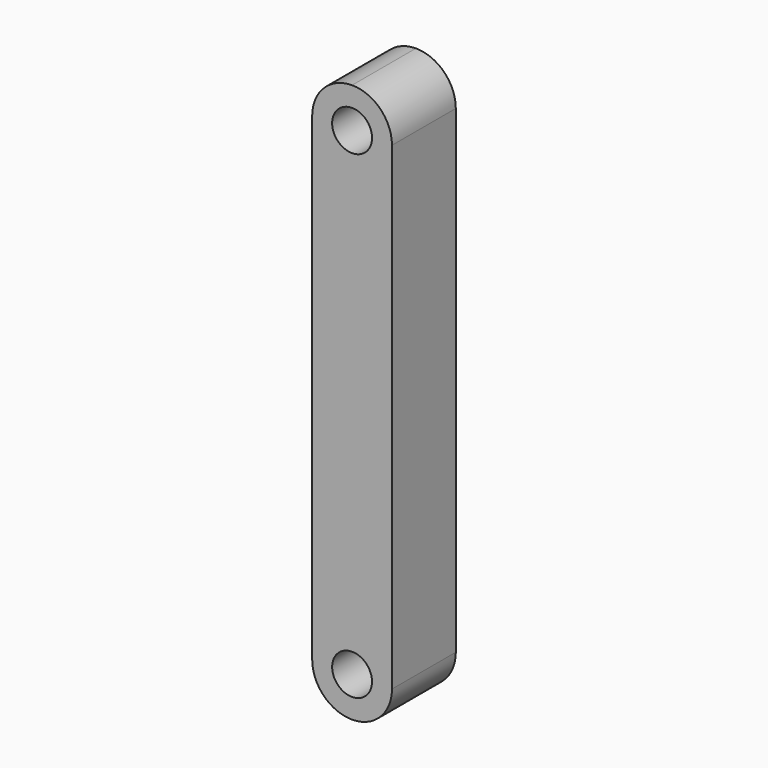
from build123d import *

# Parameters (mm, degrees)
F0_W     = 25.4
F0_H     = 177.8
F0_R     = 6.35
F1_DEPTH = 25.4
F2_R     = 12.69999


# Not quite as in the source:
# - a fillet or chamfer is up to 0.001 mm smaller than in the source, because OpenCascade refuses the exact size


with BuildPart() as f1:
    # F0 (on Front) → F1 (new body)
    with BuildSketch(Plane.XZ):
        with Locations((12.7, 88.9)):
            Rectangle(F0_W, F0_H)
        with Locations((12.7, 12.7)):
            Circle(F0_R, mode=Mode.SUBTRACT)
        with Locations((12.7, 165.1)):
            Circle(F0_R, mode=Mode.SUBTRACT)
    extrude(amount=F1_DEPTH)

    # F2 (radius 12.7 in the source; OpenCascade refuses exactly that, so slightly less here)
    f2_edges = [f1.edges().sort_by_distance(p)[0] for p in [
        (25.4, -12.7, 177.8),
        (0, -12.7, 177.8),
        (25.4, -12.7, 0),
        (0, -12.7, 0),
    ]]
    fillet(f2_edges, radius=F2_R)


solid = f1.part
